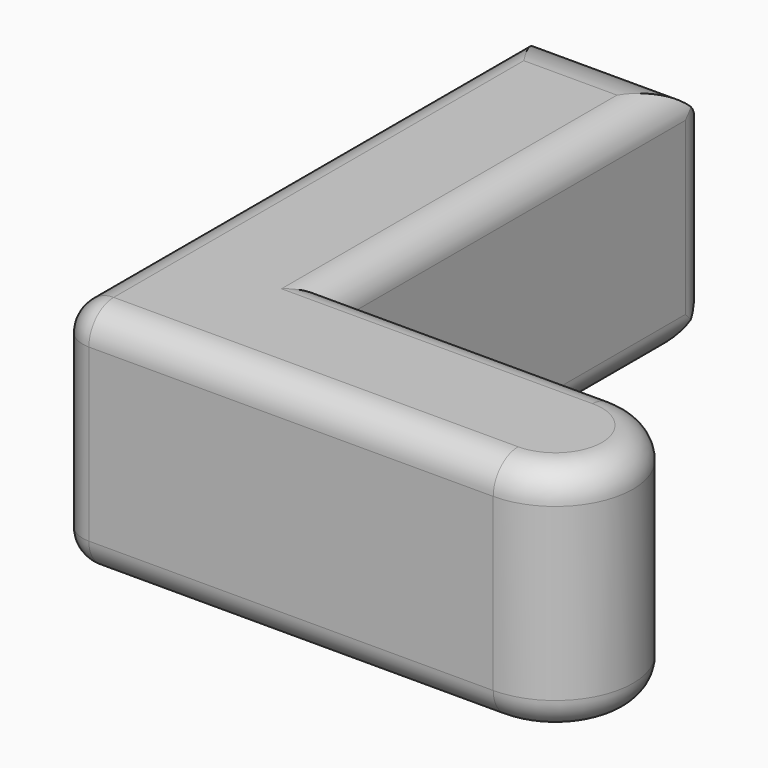
from build123d import *

# Parameters (mm, degrees)
F1_DEPTH    = 15
F2_R        = 2
F3_T1_DEPTH = 31


# Not quite as in the source:
# - a fillet or chamfer that OpenCascade refuses, or shapes differently, is made with other operations: its cross-section is extruded or revolved along the edge and cut away or added


with BuildPart() as f1:
    # F0 (on Top) → F1 (new body)
    with BuildSketch(Plane.XY):
        Polygon((0, 40), (0, 0), (28.0349999666, 0), (28.0349999666, 10), (10, 10), (10, 40), align=None)
        with BuildLine():
            Line((28.0349999666, 10), (28.0349999666, 0))
            ThreePointArc((28.0349999666, 0), (33.0349999666, 5), (28.0349999666, 10))
        make_face()
    extrude(amount=F1_DEPTH)

    # F2
    f2_edges = [f1.edges().sort_by_distance(p)[0] for p in [
        (10, 25, 15),
        (19.0175, 10, 15),
        (14.0175, 0, 0),
        (10, 40, 7.5),
        (0, 40, 7.5),
        (0, 0, 7.5),
        (0, 20, 0),
        (0, 20, 15),
        (10, 25, 0),
        (14.0175, 0, 15),
        (33.035, 5, 0),
        (33.035, 5, 15),
        (19.0175, 10, 0),
    ]]
    fillet(f2_edges, radius=F2_R)

    # F3: fillet of radius 5 on 4 edges, made by hand

    # F3_s2 → F3_t1 (cut)
    with BuildSketch(Plane.YZ.offset(-10.5)):
        with BuildLine():
            ThreePointArc((40, 5), (38.5355339059, 1.4644660941), (35, 0))
            Line((35, 0), (40, 0))
            Line((40, 0), (40, 5))
        make_face()
        with BuildLine():
            ThreePointArc((40, 10), (38.5355339059, 13.5355339059), (35, 15))
            Line((35, 15), (40, 15))
            Line((40, 15), (40, 10))
        make_face()
    extrude(amount=F3_T1_DEPTH, mode=Mode.SUBTRACT)


solid = f1.part
